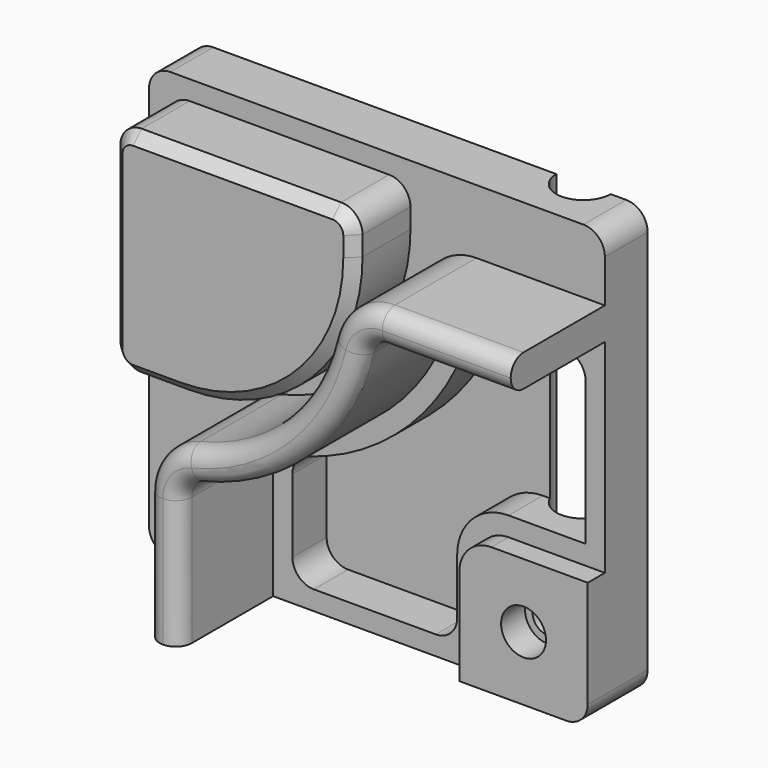
from build123d import *

# Parameters (mm, degrees)
F0_R      = 7
F1_DEPTH  = 25
F3_DEPTH  = 10
F4_R      = 10.5
F5_DEPTH  = 14
F7_DEPTH  = 55
F8_R      = 7.49999
F10_DEPTH = 20
F12_DEPTH = 33
F13_SIZE2 = 5
F13_SIZE  = 5
F15_DEPTH = 400


# Not quite as in the source:
# - a fillet or chamfer is up to 0.001 mm smaller than in the source, because OpenCascade refuses the exact size


with BuildPart() as f1:
    # F0 (on Front) → F1 (new body)
    with BuildSketch(Plane.XZ):
        with BuildLine():
            ThreePointArc((-183, -20), (-180.0710678119, -27.0710678119), (-173, -30))
            Line((-173, -30), (20, -30))
            ThreePointArc((20, -30), (27.0710678119, -27.0710678119), (30, -20))
            Line((30, -20), (30, 160))
            ThreePointArc((30, 160), (27.0710678119, 167.0710678119), (20, 170))
            Line((20, 170), (-173, 170))
            ThreePointArc((-173, 170), (-180.0710678119, 167.0710678119), (-183, 160))
            Line((-183, 160), (-183, -20))
        make_face()
        Circle(F0_R, mode=Mode.SUBTRACT)
    extrude(amount=F1_DEPTH)

    # F2 (on face) → F3 (join)
    with BuildSketch(Plane.XZ.offset(25)):
        with BuildLine():
            Line((-30, 15), (-30, -30))
            Line((-30, -30), (20, -30))
            ThreePointArc((20, -30), (27.0710678119, -27.0710678119), (30, -20))
            Line((30, -20), (30, 30))
            Line((30, 30), (-15, 30))
            ThreePointArc((-15, 30), (-25.6066017178, 25.6066017178), (-30, 15))
        make_face()
    extrude(amount=F3_DEPTH)

    # F4 (on face) → F5 (cut)
    with BuildSketch(Plane.XZ.offset(35)):
        Circle(F4_R)
    extrude(amount=-F5_DEPTH, mode=Mode.SUBTRACT)

    # F6 (on face) → F7 (join)
    with BuildSketch(Plane.XZ.offset(25)):
        with BuildLine():
            Line((-140, 30), (-140, -30))
            Line((-140, -30), (-125, -30))
            Line((-125, -30), (-125, 30))
            ThreePointArc((-125, 30), (-122.8526407389, 36.191609922), (-117.3327933147, 39.7240976625))
            ThreePointArc((-117.3327933147, 39.7240976625), (-67.5809110947, 67.5809110947), (-39.7240976625, 117.3327933147))
            ThreePointArc((-39.7240976625, 117.3327933147), (-36.191609922, 122.8526407389), (-30, 125))
            Line((-30, 125), (30, 125))
            Line((30, 125), (30, 140))
            Line((30, 140), (-30, 140))
            ThreePointArc((-30, 140), (-45.479024805, 134.6316018472), (-54.3102441564, 120.8319832868))
            ThreePointArc((-54.3102441564, 120.8319832868), (-78.1875128125, 78.1875128125), (-120.8319832868, 54.3102441564))
            ThreePointArc((-120.8319832868, 54.3102441564), (-134.6316018472, 45.479024805), (-140, 30))
        make_face()
    extrude(amount=F7_DEPTH)

    # F8 (radius 7.5 in the source; OpenCascade refuses exactly that, so slightly less here)
    f8_edges = [f1.edges().sort_by_distance(p)[0] for p in [
        (-125, -80, 0),
        (-140, -80, 0),
    ]]
    fillet(f8_edges, radius=F8_R)

    # F9 (on face) → F10 (cut)
    with BuildSketch(Plane.XZ.offset(25)):
        with BuildLine():
            ThreePointArc((-108.8892841225, 32.6891427357), (-114.0278528021, 29.0783179154), (-116, 23.1156356845))
            Line((-116, 23.1156356845), (-116, -11))
            ThreePointArc((-116, -11), (-113.0710678119, -18.0710678119), (-106, -21))
            Line((-106, -21), (-49, -21))
            ThreePointArc((-49, -21), (-41.9289321881, -18.0710678119), (-39, -11))
            Line((-39, -11), (-39, 15))
            ThreePointArc((-39, 15), (-31.9705627485, 31.9705627485), (-15, 39))
            Line((-15, 39), (21, 39))
            Line((21, 39), (21, 106))
            ThreePointArc((21, 106), (18.0710678119, 113.0710678119), (11, 116))
            Line((11, 116), (-23.1156356845, 116))
            ThreePointArc((-23.1156356845, 116), (-29.0783179154, 114.0278528021), (-32.6891427357, 108.8892841225))
            ThreePointArc((-32.6891427357, 108.8892841225), (-61.216950064, 61.216950064), (-108.8892841225, 32.6891427357))
        make_face()
    extrude(amount=-F10_DEPTH, mode=Mode.SUBTRACT)

    # F11 (on face) → F12 (join)
    with BuildSketch(Plane.XZ.offset(25)):
        with BuildLine():
            Line((-70.8271231193, 161), (-164, 161))
            ThreePointArc((-164, 161), (-171.0710678119, 158.0710678119), (-174, 151))
            Line((-174, 151), (-174, 70.8271231193))
            ThreePointArc((-174, 70.8271231193), (-171.0710678119, 63.7560553074), (-164, 60.8271231193))
            Line((-164, 60.8271231193), (-141.8271231193, 60.8271231193))
            ThreePointArc((-141.8271231193, 60.8271231193), (-84.5514738432, 84.5514738432), (-60.8271231193, 141.8271231193))
            Line((-60.8271231193, 141.8271231193), (-60.8271231193, 151))
            ThreePointArc((-60.8271231193, 151), (-63.7560553074, 158.0710678119), (-70.8271231193, 161))
        make_face()
    extrude(amount=F12_DEPTH)

    # F13
    f13_edges = [f1.edges().sort_by_distance(p)[0] for p in [
        (-174, -58, 110.913562),
    ]]
    chamfer(f13_edges, length=F13_SIZE, length2=F13_SIZE2)

    # F14 (on face) → F15 (cut)
    with BuildSketch(Plane(origin=(0, 0, -30), x_dir=(1, 0, 0), z_dir=(0, 0, -1))):
        with BuildLine():
            Line((-12.6804448871, 0), (12.6804448871, 0))
            ThreePointArc((12.6804448871, 0), (0, 12.6804448871), (-12.6804448871, 0))
        make_face()
    extrude(amount=-F15_DEPTH, mode=Mode.SUBTRACT)


solid = f1.part
